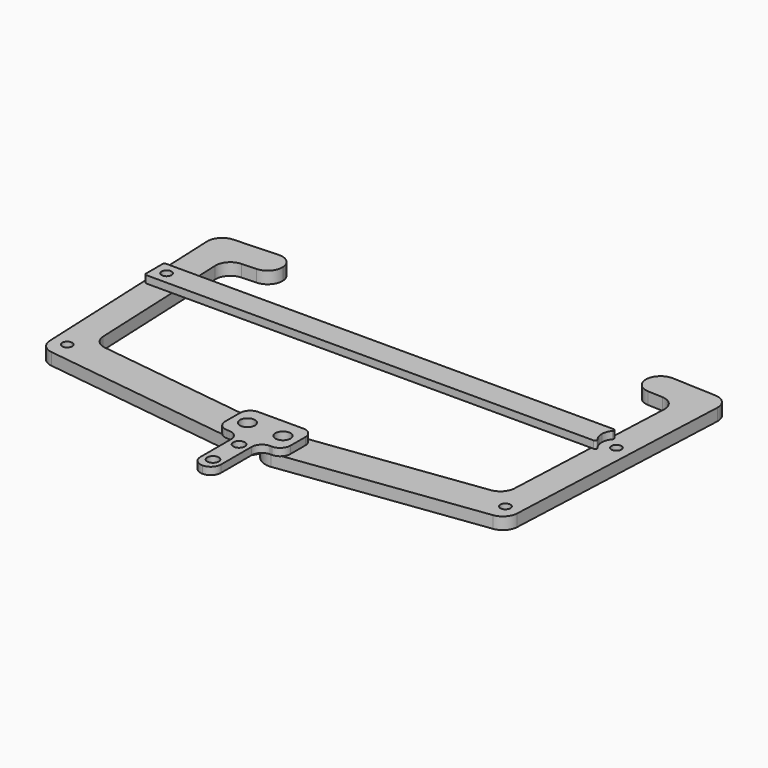
from build123d import *

# Parameters (mm, degrees)
F0_R     = 3.2512
F0_R_2   = 2.159
F1_DEPTH = 5.207
F2_R     = 3.2512
F2_W     = 8.89
F2_H     = 25.4
F2_R_2   = 2.4892
F3_DEPTH = 3.175
F4_R     = 4.44499
F5_R     = 2.159
F6_DEPTH = 3.175
F7_R     = 0.79375
F8_R     = 6.34999
F8_2_R   = 6.34999


# Not quite as in the source:
# - a fillet or chamfer is up to 0.001 mm smaller than in the source, because OpenCascade refuses the exact size


with BuildPart() as f1:
    # F0 (on Top) → F1 (new body)
    with BuildSketch(Plane.XY):
        with BuildLine():
            ThreePointArc((5.2321866987, -60.139664194), (1.4434761951, -62.9421602277), (0, -67.4282150393))
            ThreePointArc((0, -67.4282150393), (2.6205330591, -73.2118547441), (8.6967411267, -75.0550523098))
            Line((8.6967411267, -75.0550523098), (100.7307979156, -62.9385388704))
            Line((100.7307979156, -62.9385388704), (105.7164938914, 51.2526728564))
            Line((105.7164938914, 51.2526728564), (73.9967128562, 52.6375884052))
            Line((73.9967128562, 52.6375884052), (73.4427466367, 39.9496759911))
            Line((73.4427466367, 39.9496759911), (92.4746152578, 39.1187266618))
            Line((92.4746152578, 39.1187266618), (88.6202207603, -49.1614212409))
            Line((88.6202207603, -49.1614212409), (5.2321866987, -60.139664194))
        make_face()
        with Locations((7.6926489511, -67.4282150369)):
            Circle(F0_R, mode=Mode.SUBTRACT)
        with Locations((94.6755093379, -56.0499800557)):
            Circle(F0_R_2, mode=Mode.SUBTRACT)
        with Locations((97.1566728062, 0.7780063098)):
            Circle(F0_R_2, mode=Mode.SUBTRACT)
    extrude(amount=F1_DEPTH)

    # F8 (radius 6.35 in the source; OpenCascade refuses exactly that, so slightly less here)
    f8_edges = [f1.edges().sort_by_distance(p)[0] for p in [
        (92.474615, 39.118727, 2.6035),
        (73.442747, 39.949676, 2.6035),
        (73.996713, 52.637588, 2.6035),
        (105.716494, 51.252673, 2.6035),
        (100.730798, -62.938539, 2.6035),
        (88.620221, -49.161421, 2.6035),
    ]]
    fillet(f8_edges, radius=F8_R)


with BuildPart() as f1b:
    # F0 (on Top) → F1, piece 2 (new body)
    with BuildSketch(Plane.XY):
        with BuildLine():
            Line((-73.4427466367, 39.9496759911), (-105.1625276719, 38.5647604423))
            Line((-105.1625276719, 38.5647604423), (-100.7307979156, -62.9385388704))
            Line((-100.7307979156, -62.9385388704), (-8.6967411267, -75.0550523098))
            ThreePointArc((-8.6967411267, -75.0550523098), (-2.6205330591, -73.2118547441), (0, -67.4282150393))
            ThreePointArc((0, -67.4282150393), (-1.4434761951, -62.9421602277), (-5.2321866987, -60.139664194))
            Line((-5.2321866987, -60.139664194), (-88.6202207603, -49.1614212409))
            Line((-88.6202207603, -49.1614212409), (-91.9206490383, 26.4308142477))
            Line((-91.9206490383, 26.4308142477), (-72.8887804171, 27.261763577))
            Line((-72.8887804171, 27.261763577), (-73.4427466367, 39.9496759911))
        make_face()
        with Locations((-94.6755093379, -56.0499800557)):
            Circle(F0_R_2, mode=Mode.SUBTRACT)
        with Locations((-7.6926489511, -67.4282150369)):
            Circle(F0_R, mode=Mode.SUBTRACT)
        with Locations((-97.1566728062, 0.7780063098)):
            Circle(F0_R_2, mode=Mode.SUBTRACT)
    extrude(amount=F1_DEPTH)

    # F8#2 (radius 6.35 in the source; OpenCascade refuses exactly that, so slightly less here)
    f8_2_edges = [f1b.edges().sort_by_distance(p)[0] for p in [
        (-73.442747, 39.949676, 2.6035),
        (-72.88878, 27.261764, 2.6035),
        (-105.162528, 38.56476, 2.6035),
        (-91.920649, 26.430814, 2.6035),
        (-100.730798, -62.938539, 2.6035),
        (-88.620221, -49.161421, 2.6035),
    ]]
    fillet(f8_2_edges, radius=F8_2_R)


with BuildPart() as f3:
    # F2 (on face) → F3 (new body)
    with BuildSketch(Plane.XY.offset(5.207)):
        with BuildLine():
            Line((-14.1188489511, -75.8867171605), (-4.445, -75.8867171605))
            Line((-4.445, -75.8867171605), (4.445, -75.8867171605))
            Line((4.445, -75.8867171605), (14.1188489511, -75.8867171605))
            Line((14.1188489511, -75.8867171605), (14.1188489511, -58.9697129133))
            Line((14.1188489511, -58.9697129133), (-14.1188489511, -58.9697129133))
            Line((-14.1188489511, -58.9697129133), (-5.2321866987, -60.139664194))
            ThreePointArc((-5.2321866987, -60.139664194), (-0.1994884623, -69.1687304127), (-8.6967411267, -75.0550523098))
            Line((-8.6967411267, -75.0550523098), (-14.1188489511, -74.3412182725))
            Line((-14.1188489511, -74.3412182725), (-14.1188489511, -75.8867171605))
        make_face()
        with Locations((7.6926489511, -67.4282150369)):
            Circle(F2_R, mode=Mode.SUBTRACT)
        with Locations((0, -88.5867171605)):
            Rectangle(F2_W, F2_H)
        with Locations((0, -95.6225171605)):
            Circle(F2_R_2, mode=Mode.SUBTRACT)
        with Locations((0, -81.5509171605)):
            Circle(F2_R_2, mode=Mode.SUBTRACT)
        with BuildLine():
            Line((-14.1188489511, -58.9697129133), (-14.1188489511, -74.3412182725))
            Line((-14.1188489511, -74.3412182725), (-8.6967411267, -75.0550523098))
            ThreePointArc((-8.6967411267, -75.0550523098), (-0.1994884623, -69.1687304127), (-5.2321866987, -60.139664194))
            Line((-5.2321866987, -60.139664194), (-14.1188489511, -58.9697129133))
        make_face()
        with Locations((-7.6926489511, -67.4282150369)):
            Circle(F2_R, mode=Mode.SUBTRACT)
    extrude(amount=F3_DEPTH)

    # F4 (radius 4.445 in the source; OpenCascade refuses exactly that, so slightly less here)
    f4_edges = [f3.edges().sort_by_distance(p)[0] for p in [
        (-4.445, -75.886717, 6.7945),
        (-14.118849, -75.886717, 6.7945),
        (4.445, -75.886717, 6.7945),
        (14.118849, -75.886717, 6.7945),
        (14.118849, -58.969713, 6.7945),
        (-14.118849, -58.969713, 6.7945),
        (-4.445, -101.286717, 6.7945),
        (4.445, -101.286717, 6.7945),
    ]]
    fillet(f4_edges, radius=F4_R)


with BuildPart() as f6:
    # F5 (on face) → F6 (new body)
    with BuildSketch(Plane.XY.offset(5.207)):
        Polygon((90.567735786, -4.5559936902), (90.812716549, 1.0549882694), (91.0335107249, 6.1120063098), (-102.4906728062, 6.1120063098), (-102.4906728062, -4.5559936902), align=None)
        with Locations((-97.1566728062, 0.7780063098)):
            Circle(F5_R, mode=Mode.SUBTRACT)
        with BuildLine():
            ThreePointArc((93.7112491748, -4.5559936902), (91.5149736571, -2.1363942651), (90.812716549, 1.0549882694))
            Line((90.812716549, 1.0549882694), (90.567735786, -4.5559936902))
            Line((90.567735786, -4.5559936902), (93.7112491748, -4.5559936902))
        make_face()
        with BuildLine():
            ThreePointArc((90.812716549, 1.0549882694), (91.6474670997, 3.9357194829), (93.7112491748, 6.1120063098))
            Line((93.7112491748, 6.1120063098), (91.0335107249, 6.1120063098))
            Line((91.0335107249, 6.1120063098), (90.812716549, 1.0549882694))
        make_face()
    extrude(amount=F6_DEPTH)

    # F7
    f7_edges = [f6.edges().sort_by_distance(p)[0] for p in [
        (-102.490673, 6.112006, 6.7945),
        (-102.490673, -4.555994, 6.7945),
        (93.711249, 6.112006, 6.7945),
        (93.711249, -4.555994, 6.7945),
    ]]
    fillet(f7_edges, radius=F7_R)


solid = Compound([f1.part, f1b.part, f3.part, f6.part])
